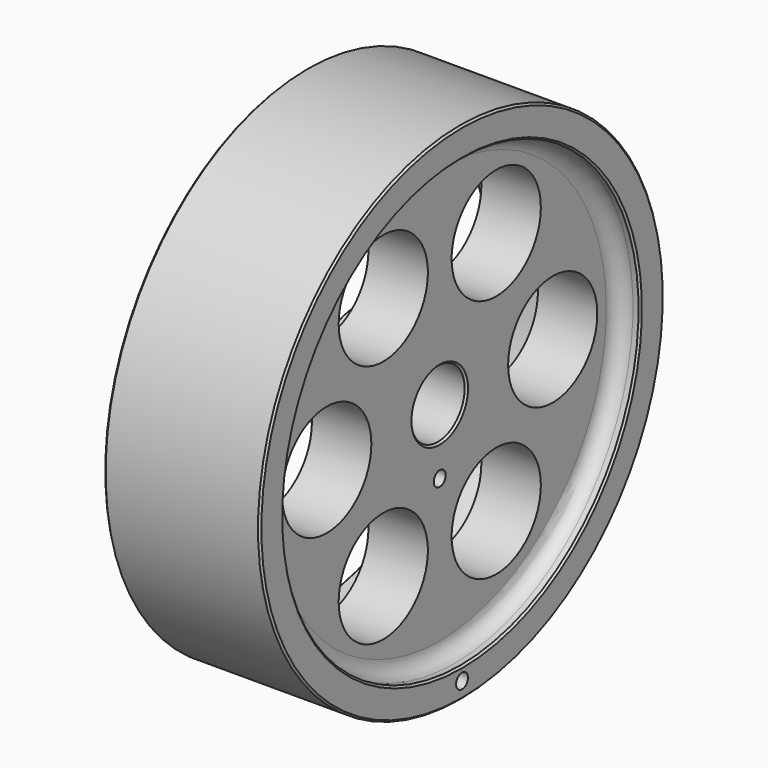
from build123d import *

# Parameters (mm, degrees)
F3_R            = 7.5
F4_DEPTH        = 12.5
F4_COPIES_COUNT = 6
F6_D            = 2
F6_DEPTH        = 7
F6_TIP          = 0.600860619


# Not quite as in the source:
# - a fillet or chamfer that OpenCascade refuses, or shapes differently, is made with other operations: its cross-section is extruded or revolved along the edge and cut away or added
# - a pattern or mirror of a feature is missing from the dataset's text; its kind, count and spacing are read off the source's solid


with BuildPart() as f1:
    # F0 (on Front) → F1 (revolve)
    with BuildSketch(Plane.XZ):
        with BuildLine():
            Line((0, 8), (0, 5))
            Line((0, 5), (11.5, 4.4978991566))
            Line((11.5, 4.4978991566), (11.5, 28))
            ThreePointArc((11.5, 28), (12.0857864376, 29.4142135624), (13.5, 30))
            Line((13.5, 30), (14.5, 30))
            Line((14.5, 30), (14.5, 34))
            Line((14.5, 34), (-6.5, 34))
            Line((-6.5, 34), (-6.5, 30))
            Line((-6.5, 30), (1.5, 30))
            ThreePointArc((1.5, 30), (2.9142135624, 29.4142135624), (3.5, 28))
            Line((3.5, 28), (3.5, 10))
            ThreePointArc((3.5, 10), (2.9142135624, 8.5857864376), (1.5, 8))
            Line((1.5, 8), (0, 8))
        make_face()
    revolve(axis=Axis((5.75, 0, 0), (1, 0, 0)))

    # F2: chamfer of 0.25 on 7 edges, made by hand

    # F2_s1 → F2_t2 (revolve, cut)
    with BuildSketch(Plane.XZ):
        Polygon((-6.25, 34), (-6.5, 33.75), (-6.5, 34), align=None)
    revolve(axis=Axis((-6.5, 0, 0), (1, 0, 0)), mode=Mode.SUBTRACT)

    # F2_s3 → F2_t4 (revolve, cut)
    with BuildSketch(Plane.XZ):
        Polygon((-6.5, 30.25), (-6.25, 30), (-6.5, 30), align=None)
    revolve(axis=Axis((-6.5, 0, 0), (1, 0, 0)), mode=Mode.SUBTRACT)

    # F2_s5 → F2_t6 (revolve, cut)
    with BuildSketch(Plane.XZ):
        Polygon((14.25, 30), (14.5, 30.25), (14.5, 30), align=None)
    revolve(axis=Axis((14.5, 0, 0), (1, 0, 0)), mode=Mode.SUBTRACT)

    # F2_s7 → F2_t8 (revolve, cut)
    with BuildSketch(Plane.XZ):
        Polygon((14.5, 33.75), (14.25, 34), (14.5, 34), align=None)
    revolve(axis=Axis((14.5, 0, 0), (1, 0, 0)), mode=Mode.SUBTRACT)

    # F2_s9 → F2_t10 (revolve, cut)
    with BuildSketch(Plane.XZ):
        Polygon((0.25, 8), (0, 7.75), (0, 8), align=None)
    revolve(axis=Axis((0, 0, 0), (1, 0, 0)), mode=Mode.SUBTRACT)

    # F2_s11 → F2_t12 (revolve, cut)
    with BuildSketch(Plane.XZ):
        Polygon((0, 5.2393229356), (0.2390951532, 4.9895608802), (0, 5), align=None)
    revolve(axis=Axis((0, 0, 0), (1, 0, 0)), mode=Mode.SUBTRACT)

    # F2_s13 → F2_t14 (revolve, cut)
    with BuildSketch(Plane.XZ):
        Polygon((11.2390951532, 4.5092905082), (11.5, 4.7590525636), (11.5, 4.4978991566), align=None)
    revolve(axis=Axis((11.5, 0, 0), (1, 0, 0)), mode=Mode.SUBTRACT)

    # F3 (on Right) → F4 (cut, symmetric)
    with BuildSketch(Plane.YZ):
        with Locations((-19, 0)):
            Circle(F3_R)
    f4 = extrude(amount=F4_DEPTH, both=True, mode=Mode.SUBTRACT)

    # F4_copies: F4 ×6 about axis
    f4_copies_axis = Axis((0, 0, 0), (1, 0, 0))
    for i in range(1, F4_COPIES_COUNT):
        add(f4.rotate(f4_copies_axis, i * 360 / F4_COPIES_COUNT), mode=Mode.SUBTRACT)

    # F6
    with Locations(Plane.YZ.offset(14.5)):
        with Locations((0, -31.75), (0, -8.75)):
            Hole(F6_D / 2, depth=F6_DEPTH)
            with Locations((0, 0, -(F6_DEPTH + F6_TIP / 2))):  # 118° drill point
                Cone(0, F6_D / 2, F6_TIP, mode=Mode.SUBTRACT)


solid = f1.part
